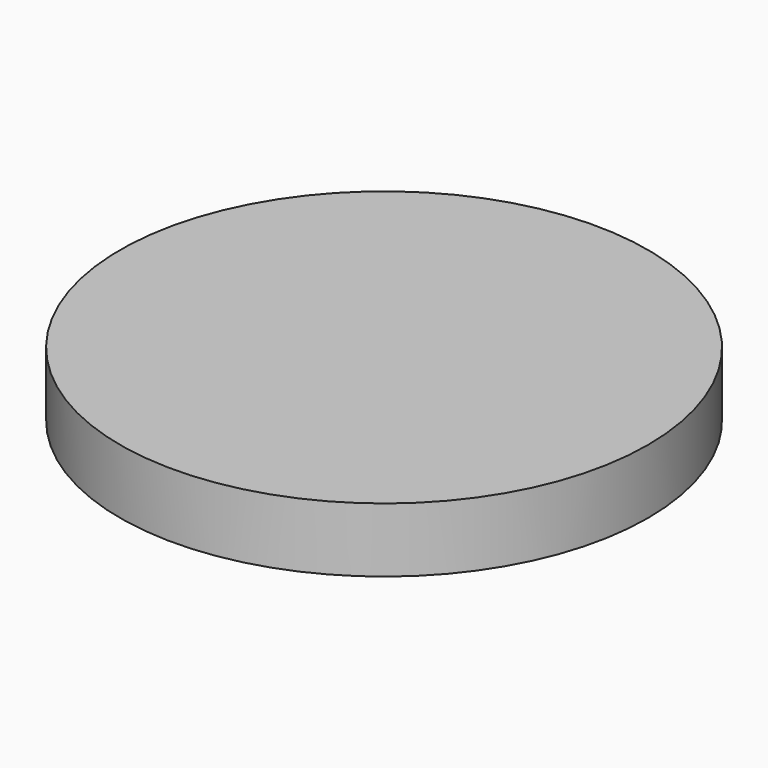
from build123d import *

# Parameters (mm, degrees)
F2_R     = 20.5
F3_DEPTH = 5


# Not quite as in the source:
# - the program builds the solid bodies; features that only make, move or delete a surface that nothing else refers to are left out


with BuildPart() as f3:
    # F2 (on Top) → F3 (new body)
    with BuildSketch(Plane.XY):
        with Locations((-46.3043488562, 17.1195659786)):
            Circle(F2_R)
    extrude(amount=F3_DEPTH)


solid = f3.part
